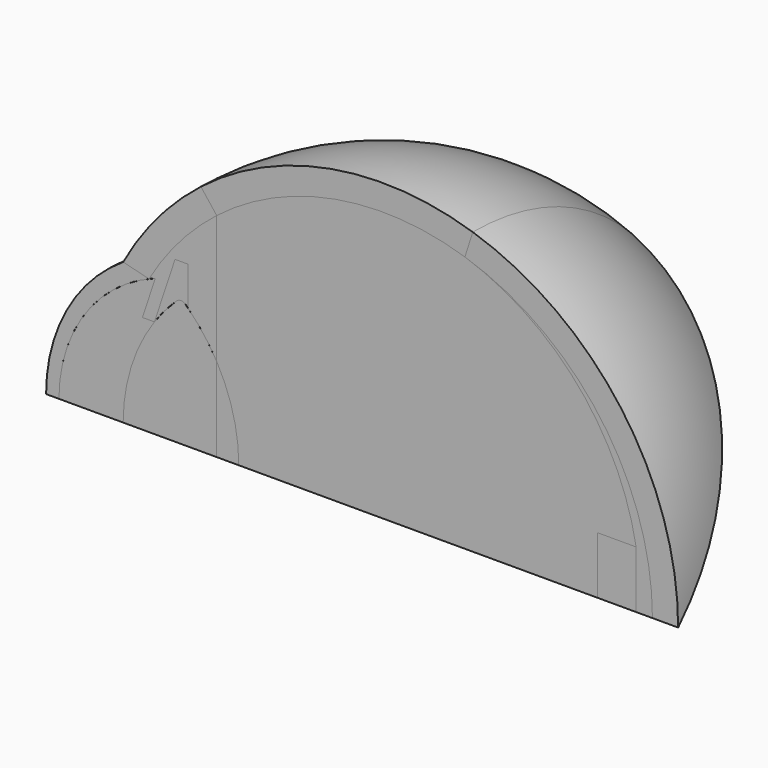
from build123d import *

# Parameters (mm, degrees)
F1_ANGLE  = 45
F3_ANGLE  = 45
F4_ANGLE  = 45
F6_ANGLE  = 45
F7_ANGLE  = 45
F9_ANGLE  = 45
F10_ANGLE = 45
F11_W     = 1.51221
F11_H     = 2.23
F12_ANGLE = 45
F13_ANGLE = 45
F15_ANGLE = 45
F16_ANGLE = 45
F19_ANGLE = 45
F22_ANGLE = 45
F25_ANGLE = 45
F28_ANGLE = 45
F31_ANGLE = 45
F34_ANGLE = 45


with BuildPart() as f1:
    # F0 (on Front) → F1 (revolve)
    with BuildSketch(Plane.XZ):
        with BuildLine():
            Line((-11.5, 0), (11.5, 0))
            ThreePointArc((11.5, 0), (2.8377537956, 11.1443776585), (-10.0995049384, 5.5))
            ThreePointArc((-10.0995049384, 5.5), (-12.3007384778, 3.1324910215), (-13.0995049384, 0))
            Line((-13.0995049384, 0), (-11.5, 0))
        make_face()
    revolve(axis=Axis((0, 0, 0), (-1, 0, 0)), revolution_arc=F1_ANGLE)

    # F2 (on Front) → F3 (revolve, cut)
    with BuildSketch(Plane.XZ):
        with BuildLine():
            ThreePointArc((11.5, 0), (2.8377537956, 11.1443776585), (-10.0995049384, 5.5))
            Line((-10.0995049384, 5.5), (-9.0932667397, 5.25))
            ThreePointArc((-9.0932667397, 5.25), (2.7175999736, 10.142221176), (10.5, 0))
            Line((10.5, 0), (11.5, 0))
        make_face()
    revolve(axis=Axis((0, 0, 0), (-1, 0, 0)), revolution_arc=F3_ANGLE, mode=Mode.SUBTRACT)

    # F5 (on face) → F6 (revolve, cut)
    with BuildSketch(Plane.XZ):
        with BuildLine():
            ThreePointArc((-12.5995049384, 0), (-11.6423500551, 3.1565885979), (-9.0932667397, 5.25))
            Line((-9.0932667397, 5.25), (-10.0995049384, 5.5))
            ThreePointArc((-10.0995049384, 5.5), (-12.3007384778, 3.1324910215), (-13.0995049384, 0))
            Line((-13.0995049384, 0), (-12.5995049384, 0))
        make_face()
    revolve(axis=Axis((-12.2997524692, 0, 0), (-1, 0, 0)), revolution_arc=F6_ANGLE, mode=Mode.SUBTRACT)

    # F8 (on Front) → F9 (revolve, cut)
    with BuildSketch(Plane.XZ):
        with BuildLine():
            ThreePointArc((3.2015621187, 10), (8.2807192075, 6.1420955145), (10, 0))
            Line((10, 0), (10.5, 0))
            ThreePointArc((10.5, 0), (8.4813442993, 6.1900564518), (3.2015621187, 10))
        make_face()
    revolve(axis=Axis((0, 0, 0), (-1, 0, 0)), revolution_arc=F9_ANGLE, mode=Mode.SUBTRACT)

    # F11 (on face) → F12 (revolve, cut)
    with BuildSketch(Plane.XZ):
        with Locations((9.1086225685, 1.115)):
            Rectangle(F11_W, F11_H)
    revolve(axis=Axis((9.1086225685, 0, 0), (-1, 0, 0)), revolution_arc=F12_ANGLE, mode=Mode.SUBTRACT)

    # F14 (on Front) → F15 (revolve, cut)
    with BuildSketch(Plane.XZ):
        with BuildLine():
            ThreePointArc((10, 0), (9.9947523902, 1.1187845105), (9.8647275685, 2.23))
            Line((9.8647275685, 2.23), (9.8647275685, 0))
            Line((9.8647275685, 0), (10, 0))
        make_face()
    revolve(axis=Axis((9.9323637842, 0, 0), (-1, 0, 0)), revolution_arc=F15_ANGLE, mode=Mode.SUBTRACT)

    # F20 (on Front) → F21 (revolve, cut)
    with BuildSketch(Plane.XZ):
        with BuildLine():
            Line((-9.3495049384, 3.8445862413), (-8.8495049384, 5.3445862413))
            ThreePointArc((-8.8495049384, 5.3445862413), (-11.5684914777, 3.2644717065), (-12.5995049384, 0))
            Line((-12.5995049384, 0), (-8.8495049384, 0))
            Line((-8.8495049384, 0), (-8.8495049384, 3.8445862413))
            Line((-8.8495049384, 3.8445862413), (-9.3495049384, 3.8445862413))
        make_face()
    revolve(axis=Axis((-10.7245049384, 0, 0), (1, 0, 0)), mode=Mode.SUBTRACT)


with BuildPart() as f4:
    # F2 (on Front) → F4 (revolve)
    with BuildSketch(Plane.XZ):
        with BuildLine():
            ThreePointArc((11.5, 0), (2.8377537956, 11.1443776585), (-10.0995049384, 5.5))
            Line((-10.0995049384, 5.5), (-9.0932667397, 5.25))
            ThreePointArc((-9.0932667397, 5.25), (2.7175999736, 10.142221176), (10.5, 0))
            Line((10.5, 0), (11.5, 0))
        make_face()
    revolve(axis=Axis((0, 0, 0), (-1, 0, 0)), revolution_arc=F4_ANGLE)

    # F17 (on Front) → F18 (revolve, cut)
    with BuildSketch(Plane.XZ):
        with BuildLine():
            ThreePointArc((11.5, 0), (9.2890913754, 6.7795856377), (3.5064727967, 10.9523809524))
            Line((3.5064727967, 10.9523809524), (3.2015621187, 10))
            ThreePointArc((3.2015621187, 10), (8.4813442993, 6.1900564518), (10.5, 0))
            Line((10.5, 0), (11.5, 0))
        make_face()
    revolve(axis=Axis((11, 0, 0), (1, 0, 0)), mode=Mode.SUBTRACT)

    # F29 (on Front) → F30 (revolve, cut)
    with BuildSketch(Plane.XZ):
        with BuildLine():
            ThreePointArc((-9.0932667397, 5.25), (-7.9222484154, 6.8911523017), (-6.4591549508, 8.2782436134))
            Line((-6.4591549508, 8.2782436134), (-7.0743125651, 9.066647767))
            ThreePointArc((-7.0743125651, 9.066647767), (-8.7701337495, 7.438733361), (-10.0995049384, 5.5))
            Line((-10.0995049384, 5.5), (-9.0932667397, 5.25))
        make_face()
    revolve(axis=Axis((-7.8495049384, 0, 0), (-1, 0, 0)), mode=Mode.SUBTRACT)


with BuildPart() as f7:
    # F5 (on face) → F7 (revolve)
    with BuildSketch(Plane.XZ):
        with BuildLine():
            ThreePointArc((-12.5995049384, 0), (-11.6423500551, 3.1565885979), (-9.0932667397, 5.25))
            Line((-9.0932667397, 5.25), (-10.0995049384, 5.5))
            ThreePointArc((-10.0995049384, 5.5), (-12.3007384778, 3.1324910215), (-13.0995049384, 0))
            Line((-13.0995049384, 0), (-12.5995049384, 0))
        make_face()
    revolve(axis=Axis((0, 0, 0), (-1, 0, 0)), revolution_arc=F7_ANGLE)


with BuildPart() as f10:
    # F8 (on Front) → F10 (revolve)
    with BuildSketch(Plane.XZ):
        with BuildLine():
            ThreePointArc((3.2015621187, 10), (8.2807192075, 6.1420955145), (10, 0))
            Line((10, 0), (10.5, 0))
            ThreePointArc((10.5, 0), (8.4813442993, 6.1900564518), (3.2015621187, 10))
        make_face()
    revolve(axis=Axis((10.25, 0, 0), (-1, 0, 0)), revolution_arc=F10_ANGLE)

    # F14 (on Front) → F16 (revolve)
    with BuildSketch(Plane.XZ):
        with BuildLine():
            ThreePointArc((10, 0), (9.9947523902, 1.1187845105), (9.8647275685, 2.23))
            Line((9.8647275685, 2.23), (9.8647275685, 0))
            Line((9.8647275685, 0), (10, 0))
        make_face()
    revolve(axis=Axis((0, 0, 0), (-1, 0, 0)), revolution_arc=F16_ANGLE)


with BuildPart() as f13:
    # F11 (on face) → F13 (revolve)
    with BuildSketch(Plane.XZ):
        with Locations((9.1086225685, 1.115)):
            Rectangle(F11_W, F11_H)
    revolve(axis=Axis((0, 0, 0), (-1, 0, 0)), revolution_arc=F13_ANGLE)


with BuildPart() as f19:
    # F17 (on Front) → F19 (revolve)
    with BuildSketch(Plane.XZ):
        with BuildLine():
            ThreePointArc((11.5, 0), (9.2890913754, 6.7795856377), (3.5064727967, 10.9523809524))
            Line((3.5064727967, 10.9523809524), (3.2015621187, 10))
            ThreePointArc((3.2015621187, 10), (8.4813442993, 6.1900564518), (10.5, 0))
            Line((10.5, 0), (11.5, 0))
        make_face()
    revolve(axis=Axis((0, 0, 0), (-1, 0, 0)), revolution_arc=F19_ANGLE)


with BuildPart() as f22:
    # F20 (on Front) → F22 (revolve)
    with BuildSketch(Plane.XZ):
        with BuildLine():
            Line((-9.3495049384, 3.8445862413), (-8.8495049384, 5.3445862413))
            ThreePointArc((-8.8495049384, 5.3445862413), (-11.5684914777, 3.2644717065), (-12.5995049384, 0))
            Line((-12.5995049384, 0), (-8.8495049384, 0))
            Line((-8.8495049384, 0), (-8.8495049384, 3.8445862413))
            Line((-8.8495049384, 3.8445862413), (-9.3495049384, 3.8445862413))
        make_face()
    revolve(axis=Axis((0, 0, 0), (-1, 0, 0)), revolution_arc=F22_ANGLE)


with BuildPart() as f24_tool:
    # F23 (on Front) → F24 (revolve)
    with BuildSketch(Plane.XZ):
        with BuildLine():
            Line((-10.0995049384, 0), (-5.5995049384, 0))
            ThreePointArc((-5.5995049384, 0), (-6.1408791354, 2.6344401261), (-7.6772587181, 4.8419044128))
            ThreePointArc((-7.6772587181, 4.8419044128), (-7.8495049384, 4.9107104847), (-8.0217511587, 4.8419044128))
            ThreePointArc((-8.0217511587, 4.8419044128), (-9.5581307413, 2.6344401261), (-10.0995049384, 0))
        make_face()
    revolve(axis=Axis((0, 0, 0), (-1, 0, 0)))


with BuildPart() as f1_1:
    add(f1.part)

    # F24: cut by f24_tool
    add(f24_tool.part, mode=Mode.SUBTRACT)

    # F26 (on Front) → F27 (revolve, cut)
    with BuildSketch(Plane.XZ):
        with BuildLine():
            Line((-8.8495049384, 5.3445862413), (-9.3495049384, 3.8445862413))
            Line((-9.3495049384, 3.8445862413), (-8.8823713109, 3.8445862413))
            Line((-8.8823713109, 3.8445862413), (-8.0810395972, 6.2485813822))
            Line((-8.0810395972, 6.2485813822), (-7.5810395972, 6.2485813822))
            Line((-7.5810395972, 6.2485813822), (-7.5810395972, 4.7485813822))
            ThreePointArc((-7.5810395972, 4.7485813822), (-6.9689696113, 4.0524234931), (-6.4591549508, 3.2782436134))
            Line((-6.4591549508, 3.2782436134), (-6.4591549508, 8.2782436134))
            ThreePointArc((-6.4591549508, 8.2782436134), (-7.9222484154, 6.8911523017), (-9.0932667397, 5.25))
            ThreePointArc((-9.0932667397, 5.25), (-8.9719298306, 5.298695062), (-8.8495049384, 5.3445862413))
        make_face()
    revolve(axis=Axis((-7.8495049384, 0, 0), (-1, 0, 0)), mode=Mode.SUBTRACT)


with BuildPart() as f22_1:
    add(f22.part)

    # F24: cut by f24_tool
    add(f24_tool.part, mode=Mode.SUBTRACT)


with BuildPart() as f25:
    # F23 (on Front) → F25 (revolve)
    with BuildSketch(Plane.XZ):
        with BuildLine():
            Line((-10.0995049384, 0), (-5.5995049384, 0))
            ThreePointArc((-5.5995049384, 0), (-6.1408791354, 2.6344401261), (-7.6772587181, 4.8419044128))
            ThreePointArc((-7.6772587181, 4.8419044128), (-7.8495049384, 4.9107104847), (-8.0217511587, 4.8419044128))
            ThreePointArc((-8.0217511587, 4.8419044128), (-9.5581307413, 2.6344401261), (-10.0995049384, 0))
        make_face()
    revolve(axis=Axis((0, 0, 0), (-1, 0, 0)), revolution_arc=F25_ANGLE)

    # F32 (on Front) → F33 (revolve, cut)
    with BuildSketch(Plane.XZ):
        with BuildLine():
            Line((-6.4591549508, 3.2782436134), (-6.4591549508, 0))
            Line((-6.4591549508, 0), (-5.5995049384, 0))
            ThreePointArc((-5.5995049384, 0), (-5.8179901834, 1.6945411866), (-6.4591549508, 3.2782436134))
        make_face()
    revolve(axis=Axis((-6.0293299446, 0, 0), (1, 0, 0)), mode=Mode.SUBTRACT)


with BuildPart() as f28:
    # F26 (on Front) → F28 (revolve)
    with BuildSketch(Plane.XZ):
        with BuildLine():
            Line((-8.8495049384, 5.3445862413), (-9.3495049384, 3.8445862413))
            Line((-9.3495049384, 3.8445862413), (-8.8823713109, 3.8445862413))
            Line((-8.8823713109, 3.8445862413), (-8.0810395972, 6.2485813822))
            Line((-8.0810395972, 6.2485813822), (-7.5810395972, 6.2485813822))
            Line((-7.5810395972, 6.2485813822), (-7.5810395972, 4.7485813822))
            ThreePointArc((-7.5810395972, 4.7485813822), (-6.9689696113, 4.0524234931), (-6.4591549508, 3.2782436134))
            Line((-6.4591549508, 3.2782436134), (-6.4591549508, 8.2782436134))
            ThreePointArc((-6.4591549508, 8.2782436134), (-7.9222484154, 6.8911523017), (-9.0932667397, 5.25))
            ThreePointArc((-9.0932667397, 5.25), (-8.9719298306, 5.298695062), (-8.8495049384, 5.3445862413))
        make_face()
    revolve(axis=Axis((-7.8495049384, 0, 0), (-1, 0, 0)), revolution_arc=F28_ANGLE)


with BuildPart() as f31:
    # F29 (on Front) → F31 (revolve)
    with BuildSketch(Plane.XZ):
        with BuildLine():
            ThreePointArc((-9.0932667397, 5.25), (-7.9222484154, 6.8911523017), (-6.4591549508, 8.2782436134))
            Line((-6.4591549508, 8.2782436134), (-7.0743125651, 9.066647767))
            ThreePointArc((-7.0743125651, 9.066647767), (-8.7701337495, 7.438733361), (-10.0995049384, 5.5))
            Line((-10.0995049384, 5.5), (-9.0932667397, 5.25))
        make_face()
    revolve(axis=Axis((-7.8495049384, 0, 0), (-1, 0, 0)), revolution_arc=F31_ANGLE)


with BuildPart() as f34:
    # F32 (on Front) → F34 (revolve)
    with BuildSketch(Plane.XZ):
        with BuildLine():
            Line((-6.4591549508, 3.2782436134), (-6.4591549508, 0))
            Line((-6.4591549508, 0), (-5.5995049384, 0))
            ThreePointArc((-5.5995049384, 0), (-5.8179901834, 1.6945411866), (-6.4591549508, 3.2782436134))
        make_face()
    revolve(axis=Axis((-7.8495049384, 0, 0), (-1, 0, 0)), revolution_arc=F34_ANGLE)


solid = Compound([f4.part, f7.part, f10.part, f13.part, f19.part, f1_1.part, f22_1.part, f25.part, f28.part, f31.part, f34.part])
